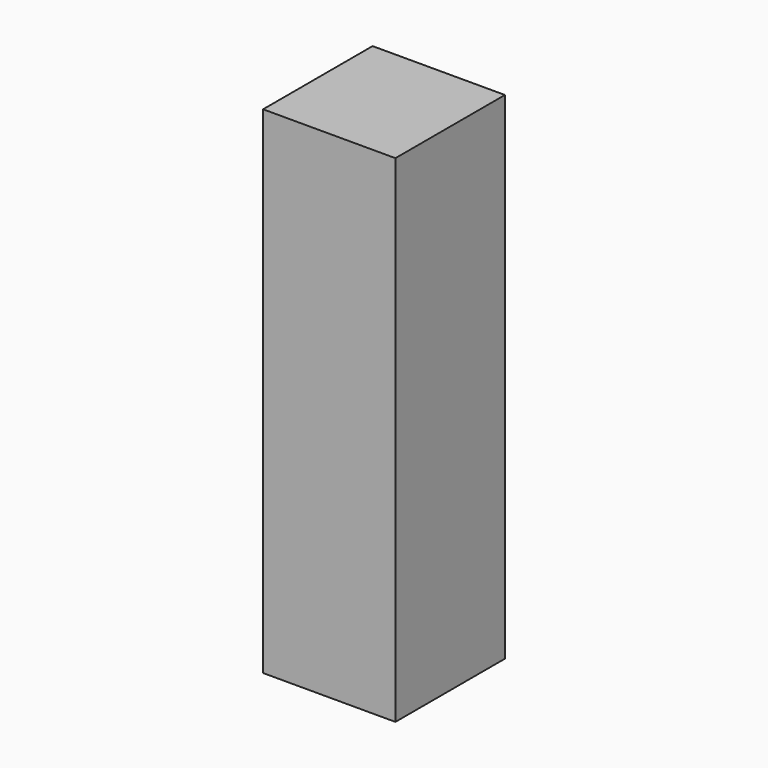
from build123d import *

# Parameters (mm, degrees)
F0_W     = 40.6355857849
F0_H     = 42.0261397958
F5_DEPTH = 152.4


# Not quite as in the source:
# - the program builds the solid bodies; features that only make, move or delete a surface that nothing else refers to are left out


with BuildPart() as f5:
    # F0 (on Top) → F5 (new body)
    with BuildSketch(Plane.XY):
        Rectangle(F0_W, F0_H)
    extrude(amount=F5_DEPTH)


solid = f5.part
